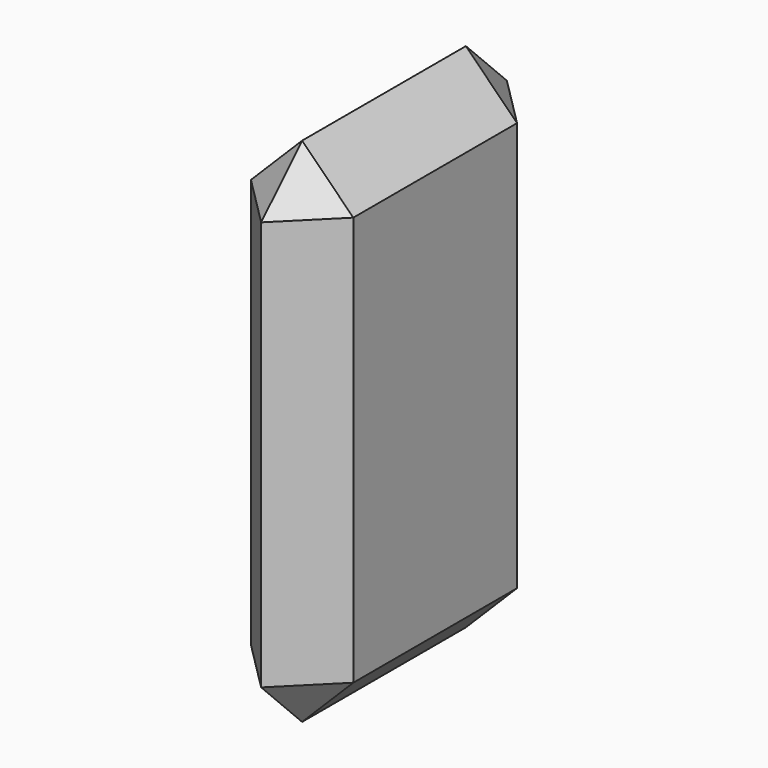
from build123d import *

# Parameters (mm, degrees)
F0_W     = 30
F0_H     = 50
F1_DEPTH = 10
F2_SIZE  = 4.99999


# Not quite as in the source:
# - a fillet or chamfer is up to 0.001 mm smaller than in the source, because OpenCascade refuses the exact size


with BuildPart() as f1:
    # F0 (on Right) → F1 (new body)
    with BuildSketch(Plane.YZ):
        Rectangle(F0_W, F0_H)
    extrude(amount=F1_DEPTH)

    # F2 (size 5 in the source; OpenCascade refuses exactly that, so slightly less here)
    f2_edges = [f1.edges().sort_by_distance(p)[0] for p in [
        (5, -15, 25),
        (5, -15, -25),
        (0, -15, 0),
        (10, -15, 0),
        (5, 15, -25),
        (5, 15, 25),
        (0, 15, 0),
        (10, 15, 0),
        (10, 0, 25),
        (10, 0, -25),
        (0, 0, 25),
        (0, 0, -25),
    ]]
    chamfer(f2_edges, length=F2_SIZE)


solid = f1.part
